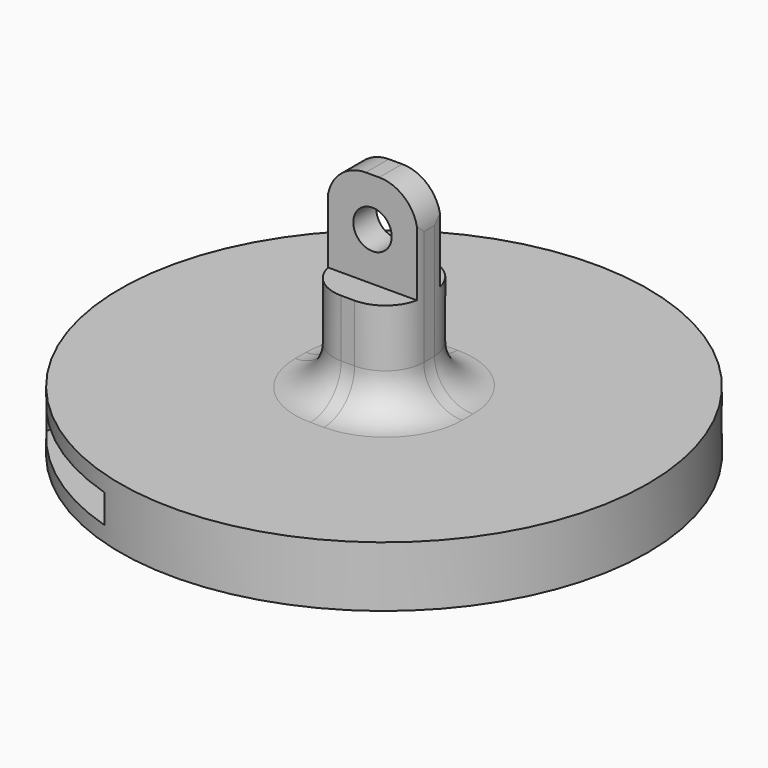
from build123d import *

# Parameters (mm, degrees)
F1_R         = 27.5
F2_DEPTH     = 6.3
F3_W         = 9.4
F3_H         = 9.4
F4_DEPTH     = 10
F5_W         = 9.4
F5_H         = 3
F6_DEPTH     = 10
F7_R         = 2
F8_DEPTH     = 25
F9_R         = 4
F10_T1_DEPTH = 20
F11_R        = 4
F12_W        = 14
F12_H        = 3
F13_DEPTH    = 25
F14_W        = 14
F14_H        = 3
F15_DEPTH    = 25


# Not quite as in the source:
# - a fillet or chamfer that OpenCascade refuses, or shapes differently, is made with other operations: its cross-section is extruded or revolved along the edge and cut away or added


with BuildPart() as f2:
    # F1 (on offset) → F2 (new body)
    with BuildSketch(Plane.XY.offset(3.6)):
        Circle(F1_R)
    extrude(amount=F2_DEPTH)

    # F3 (on face) → F4 (join)
    with BuildSketch(Plane.XY.offset(9.9)):
        Rectangle(F3_W, F3_H)
    extrude(amount=F4_DEPTH)

    # F5 (on face) → F6 (join)
    with BuildSketch(Plane.XY.offset(19.9)):
        Rectangle(F5_W, F5_H)
    extrude(amount=F6_DEPTH)

    # F7 (on face) → F8 (cut)
    with BuildSketch(Plane.XZ.offset(1.5)):
        with Locations((0, 24.9)):
            Circle(F7_R)
    extrude(amount=-F8_DEPTH, mode=Mode.SUBTRACT)

    # F9
    f9_edges = [f2.edges().sort_by_distance(p)[0] for p in [
        (-4.7, 0, 29.9),
        (4.7, 0, 29.9),
    ]]
    fillet(f9_edges, radius=F9_R)

    # F10: fillet of radius 4 on 4 edges, made by hand

    # F10_s2 → F10_t1 (cut)
    with BuildSketch(Plane.XY.offset(9.9)):
        with BuildLine():
            ThreePointArc((-0.7, -4.7), (-3.5284271247, -3.5284271247), (-4.7, -0.7))
            Line((-4.7, -0.7), (-4.7, -4.7))
            Line((-4.7, -4.7), (-0.7, -4.7))
        make_face()
        with BuildLine():
            ThreePointArc((-0.7, 4.7), (-3.5284271247, 3.5284271247), (-4.7, 0.7))
            Line((-4.7, 0.7), (-4.7, 4.7))
            Line((-4.7, 4.7), (-0.7, 4.7))
        make_face()
        with BuildLine():
            ThreePointArc((4.7, -0.7), (3.5284271247, -3.5284271247), (0.7, -4.7))
            Line((0.7, -4.7), (4.7, -4.7))
            Line((4.7, -4.7), (4.7, -0.7))
        make_face()
        with BuildLine():
            ThreePointArc((4.7, 0.7), (3.5284271247, 3.5284271247), (0.7, 4.7))
            Line((0.7, 4.7), (4.7, 4.7))
            Line((4.7, 4.7), (4.7, 0.7))
        make_face()
    extrude(amount=F10_T1_DEPTH, mode=Mode.SUBTRACT)

    # F11
    f11_edges = [f2.edges().sort_by_distance(p)[0] for p in [
        (-3.528427, -3.528427, 9.9),
    ]]
    fillet(f11_edges, radius=F11_R)

    # F12 (on face) → F13 (cut)
    with BuildSketch(Plane(origin=(0, 4.7, 0), x_dir=(-1, 0, 0), z_dir=(0, 1, 0))):
        with Locations((-15.4635200504, 6.6790340934)):
            Rectangle(F12_W, F12_H)
    extrude(amount=F13_DEPTH, mode=Mode.SUBTRACT)

    # F14 (on face) → F15 (cut)
    with BuildSketch(Plane.XZ.offset(4.7)):
        with Locations((-15.1143019667, 6.7091025412)):
            Rectangle(F14_W, F14_H)
    extrude(amount=F15_DEPTH, mode=Mode.SUBTRACT)


solid = f2.part
